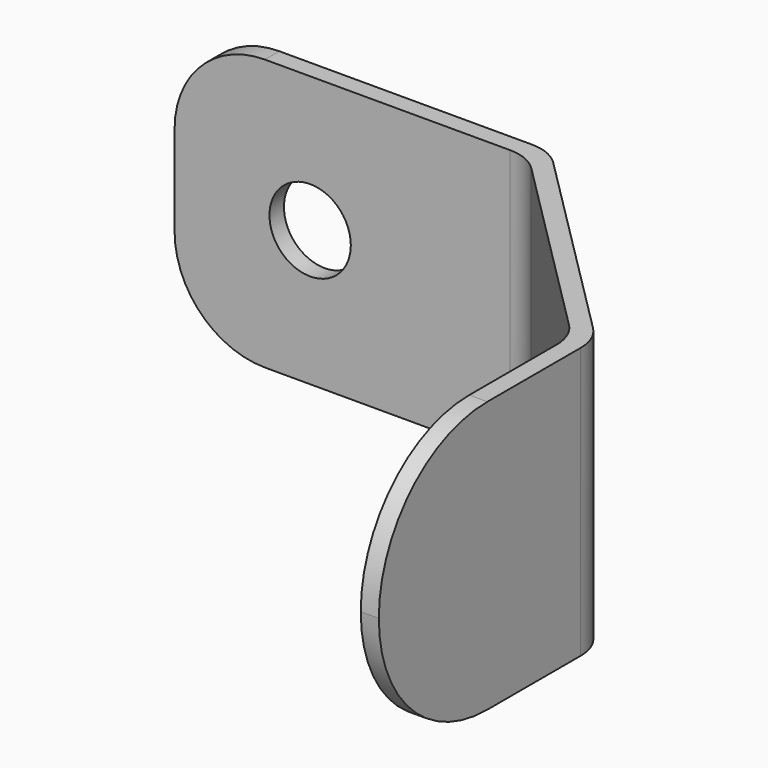
from build123d import *

# Parameters (mm, degrees)
F1_DEPTH = 15
F2_R     = 14.99999
F3_R     = 4.5
F4_DEPTH = 2.001
F5_R     = 10


# Not quite as in the source:
# - a fillet or chamfer is up to 0.001 mm smaller than in the source, because OpenCascade refuses the exact size


with BuildPart() as f1:
    # F0 (on Top) → F1 (new body, symmetric)
    with BuildSketch(Plane.XY):
        with BuildLine():
            ThreePointArc((-98.5355339059, -1.4644660941), (-100.15765065, -0.3806023374), (-102.0710678119, 0))
            Line((-102.0710678119, 0), (-140, 0))
            Line((-140, 0), (-140, -2))
            Line((-140, -2), (-102.8994949366, -2))
            ThreePointArc((-102.8994949366, -2), (-100.9860777748, -2.3806023374), (-99.3639610307, -3.4644660941))
            Line((-99.3639610307, -3.4644660941), (-78.4644660941, -24.3639610307))
            ThreePointArc((-78.4644660941, -24.3639610307), (-77.3806023374, -25.9860777748), (-77, -27.8994949366))
            Line((-77, -27.8994949366), (-77, -55))
            Line((-77, -55), (-75, -55))
            Line((-75, -55), (-75, -27.0710678119))
            ThreePointArc((-75, -27.0710678119), (-75.3806023374, -25.15765065), (-76.4644660941, -23.5355339059))
            Line((-76.4644660941, -23.5355339059), (-98.5355339059, -1.4644660941))
        make_face()
    extrude(amount=F1_DEPTH, both=True)

    # F2 (radius 15 in the source; OpenCascade refuses exactly that, so slightly less here)
    f2_edges = [f1.edges().sort_by_distance(p)[0] for p in [
        (-76, -55, 15),
        (-76, -55, -15),
    ]]
    fillet(f2_edges, radius=F2_R)

    # F3 (on face) → F4 (cut, through all)
    with BuildSketch(Plane.XZ.offset(2)):
        with Locations((-125, 0)):
            Circle(F3_R)
    extrude(amount=-F4_DEPTH, mode=Mode.SUBTRACT)

    # F5
    f5_edges = [f1.edges().sort_by_distance(p)[0] for p in [
        (-140, -1, 15),
        (-140, -1, -15),
    ]]
    fillet(f5_edges, radius=F5_R)


solid = f1.part
